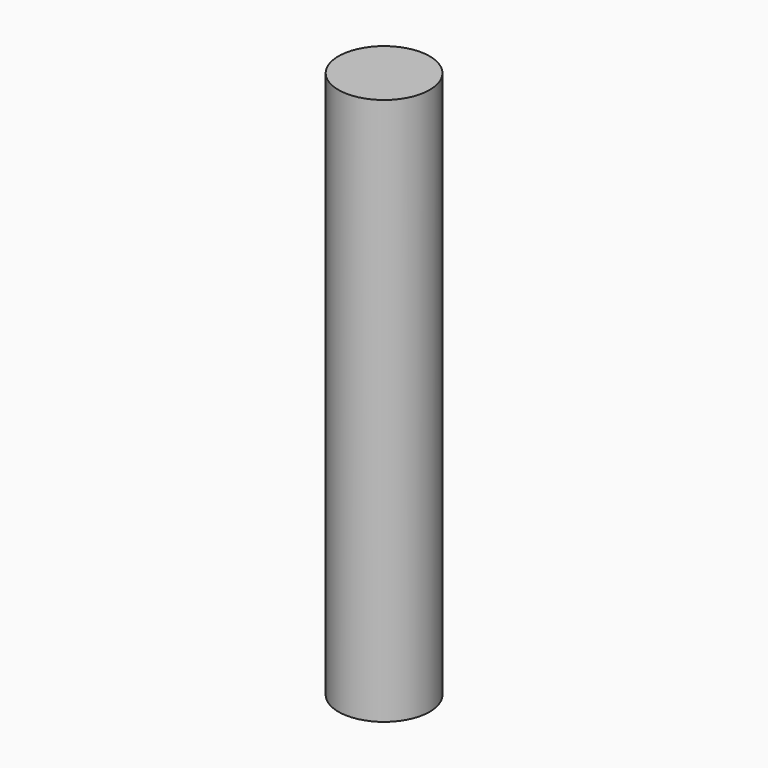
from build123d import *

# Parameters (mm, degrees)
F0_R     = 1.5875
F1_DEPTH = 19.05


# Not quite as in the source:
# - a length typed as a fraction of an inch, garbled in the dataset ("3 / 203.2 mm" for 3/8 in), is restored


with BuildPart() as f1:
    # F0 (on Top) → F1 (new body)
    with BuildSketch(Plane.XY):
        Circle(F0_R)
    extrude(amount=F1_DEPTH)


solid = f1.part
